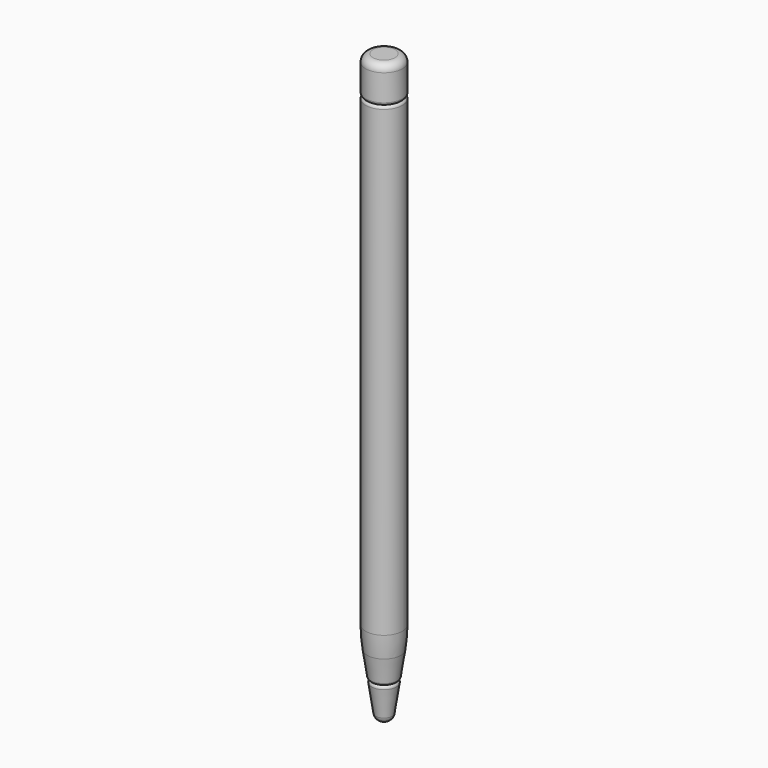
from build123d import *

# Parameters (mm, degrees)
F0_W   = 3.175
F0_H   = 6.35
F3_R   = 0.508
F3_2_R = 0.508
F3_3_R = 0.508
F4_R   = 1.27
F4_2_R = 1.27
F5_R   = 25.4


with BuildPart() as f1:
    # F0 (on Front) → F1 (revolve)
    with BuildSketch(Plane.XZ):
        Polygon((3.175, 95.25), (0, 95.25), (0, 6.35), (2.2225, 6.35), (3.175, 12.7), align=None)
    revolve(axis=Axis((0, 0, 50.8), (0, 0, -1)))

    # F3
    f3_edges = [f1.edges().sort_by_distance(p)[0] for p in [
        (-2.2225, 0, 6.35),
        (-3.175, 0, 95.25),
    ]]
    fillet(f3_edges, radius=F3_R)

    # F5
    f5_edges = [f1.edges().sort_by_distance(p)[0] for p in [
        (-3.175, 0, 12.7),
    ]]
    fillet(f5_edges, radius=F5_R)


with BuildPart() as f2:
    # F0 (on Front) → F2 (revolve)
    with BuildSketch(Plane.XZ):
        with Locations((1.5875, 98.425)):
            Rectangle(F0_W, F0_H)
    revolve(axis=Axis((0, 0, 50.8), (0, 0, -1)))

    # F3#3
    f3_3_edges = [f2.edges().sort_by_distance(p)[0] for p in [
        (-3.175, 0, 95.25),
    ]]
    fillet(f3_3_edges, radius=F3_3_R)

    # F4
    f4_edges = [f2.edges().sort_by_distance(p)[0] for p in [
        (-3.175, 0, 101.6),
    ]]
    fillet(f4_edges, radius=F4_R)


with BuildPart() as f2b:
    # F0 (on Front) → F2, piece 2 (revolve)
    with BuildSketch(Plane.XZ):
        Polygon((2.2225, 6.35), (0, 6.35), (0, 0), (1.27, 0), align=None)
    revolve(axis=Axis((0, 0, 50.8), (0, 0, -1)))

    # F3#2
    f3_2_edges = [f2b.edges().sort_by_distance(p)[0] for p in [
        (-2.2225, 0, 6.35),
    ]]
    fillet(f3_2_edges, radius=F3_2_R)

    # F4#2
    f4_2_edges = [f2b.edges().sort_by_distance(p)[0] for p in [
        (-1.27, 0, 0),
    ]]
    fillet(f4_2_edges, radius=F4_2_R)


solid = Compound([f1.part, f2.part, f2b.part])
